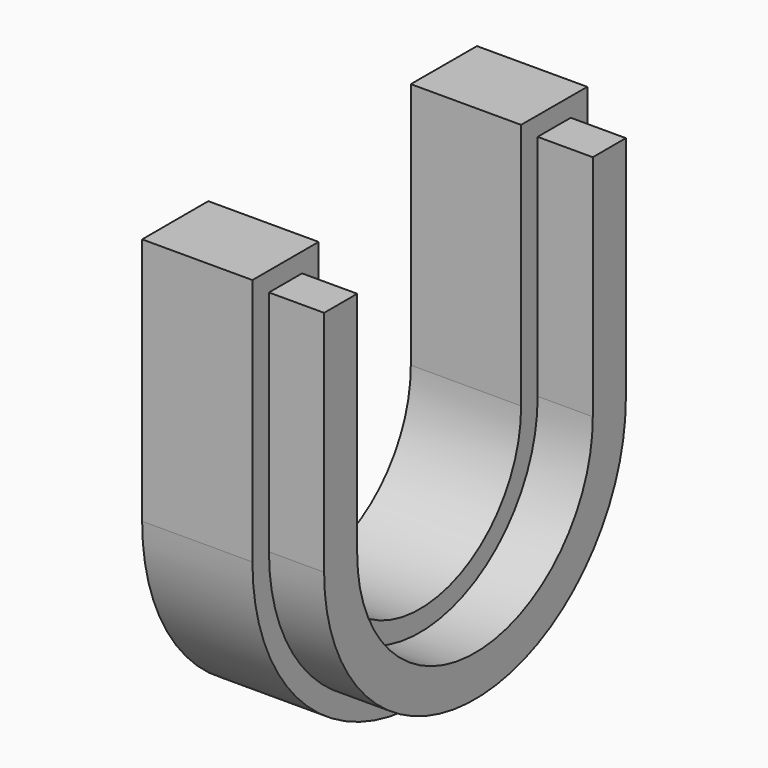
from build123d import *

# Parameters (mm, degrees)
F1_DEPTH = 25.4
F3_DEPTH = 12.7


# Not quite as in the source:
# - ends of sketch curves that miss each other by under 0.0002 mm in the source are joined


with BuildPart() as f1:
    # F0 (on Right) → F1 (new body)
    with BuildSketch(Plane.YZ):
        with BuildLine():
            Line((-28.3121045191, 76.1390224734), (-47.3621045191, 76.1390224734))
            Line((-47.3621045191, 76.1390224734), (-47.3621045191, 18.9890224734))
            ThreePointArc((-47.3621045191, 18.9890224734), (0.8307135418, -29.2037957052), (49.0235318381, 18.9890222381))
            Line((49.0235318381, 18.9890222381), (49.0235318381, 76.1390222381))
            Line((49.0235318381, 76.1390222381), (29.9735318381, 76.1725883931))
            Line((29.9735318381, 76.1725883931), (29.9735318381, 19.1909559071))
            ThreePointArc((29.9735318381, 19.1909559071), (0.9320306114, -10.1539702583), (-28.3121045191, 18.9890228212))
            Line((-28.3121045191, 18.9890228212), (-28.3121045191, 76.1390224734))
        make_face()
    extrude(amount=F1_DEPTH)


with BuildPart() as f3:
    # F2 (on face) → F3 (new body)
    with BuildSketch(Plane.YZ.offset(25.4)):
        with BuildLine():
            Line((-33.0746045191, 71.6940224734), (-42.5996045191, 71.6940224734))
            Line((-42.5996045191, 71.6940224734), (-42.5996045191, 19.1180334417))
            ThreePointArc((-42.5996045191, 19.1180334417), (0.8307136595, -24.3122847369), (44.2610318381, 19.1180334417))
            Line((44.2610318381, 19.1180334417), (44.2610318381, 71.8052499411))
            Line((44.2610318381, 71.8052499411), (34.7360318381, 71.8052499411))
            Line((34.7360318381, 71.8052499411), (34.7360318381, 19.1909559071))
            ThreePointArc((34.7360318381, 19.1909559071), (0.931981493, -14.9164460393), (-33.0746045191, 18.9890224734))
            Line((-33.0746045191, 18.9890224734), (-33.0746045191, 71.6940224734))
        make_face()
    extrude(amount=F3_DEPTH)


solid = Compound([f1.part, f3.part])
